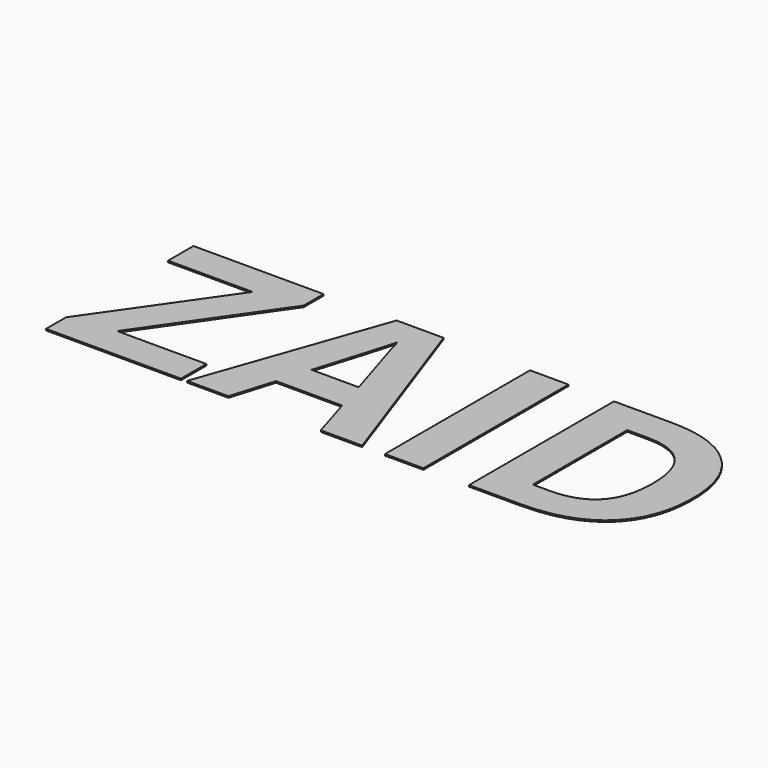
from build123d import *

# Parameters (mm, degrees)
F0_TEXT_SIZE = 21.6429237119
F1_DEPTH     = 0.127


# Not quite as in the source:
# - Text() gives the source's letters only with a copy of the font that has no kerning and outlines rounded to 1/6400 em; it was checked with that copy


with BuildPart() as f1:
    # F0 (on Top) → F1 (new body)
    with BuildSketch(Plane.XY):
        with Locations((0, 0)):
            Text('ZAID', F0_TEXT_SIZE, font='Open Sans', font_style=FontStyle.BOLD, text_align=(TextAlign.LEFT, TextAlign.BOTTOM))
    extrude(amount=F1_DEPTH)


solid = f1.part
